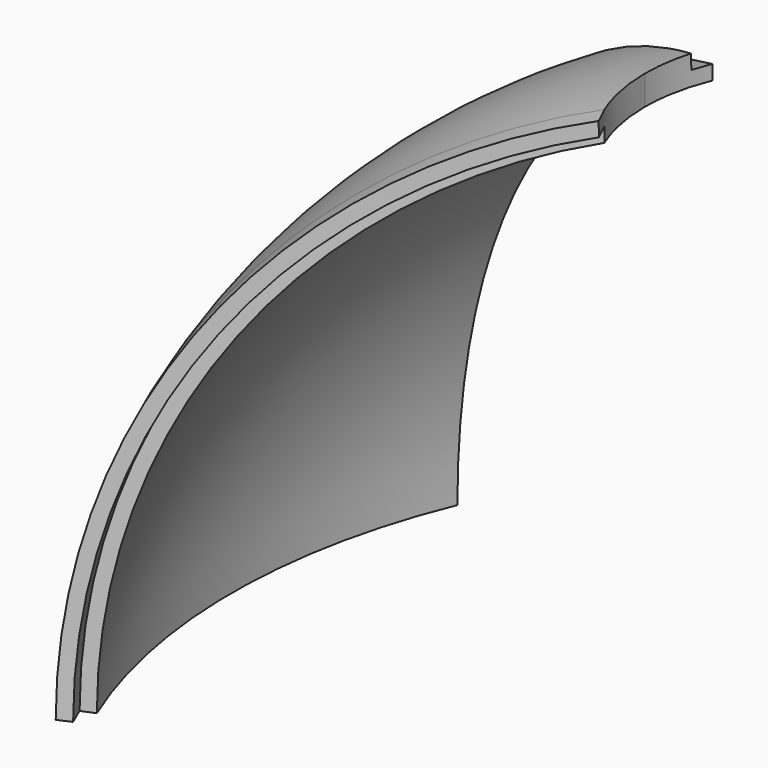
from build123d import *
from build123d import SkipClean  # not in build123d's __all__

# Parameters (mm, degrees)
F3_ANGLE_BACK = 22.5
F3_ANGLE      = 45
F8_W          = 1100
F8_H          = 4000


with BuildPart() as f3:
    # F2 (on Front) → F3 (revolve)
    with BuildSketch(Plane.XZ, mode=Mode.PRIVATE) as f3_sk:
        with BuildLine():
            Line((-1000, 3536.3293115885), (-1000, 3717.8622890043))
            ThreePointArc((-1000, 3717.8622890043), (-3055.5277776515, 2342.2745355743), (-3850, 0))
            Line((-3850, 0), (-3675, 0))
            ThreePointArc((-3675, 0), (-2930.9234892777, 2217.050405381), (-1000, 3536.3293115885))
        make_face()
    revolve(f3_sk.sketch.rotate(Axis((0, 0, 3762.5), (0, 0, 1)), -F3_ANGLE_BACK), axis=Axis((0, 0, 3762.5), (0, 0, 1)), revolution_arc=F3_ANGLE)

    # F5: sweep along a path in F5_path
    with BuildLine(Plane(origin=(-3556.9362001685, 1473.3312146056, 0), x_dir=(-0.9238795325, 0.3826834324, 0), z_dir=(-0.3826834324, -0.9238795325, 0))) as f5_path:
        ThreePointArc((0, 0), (-794.4722223485, -2342.2745355743), (-2850, -3717.8622890043))
    # F4 (on face) → F5 (sweep, cut)
    with BuildSketch(Plane(origin=(0, 0, 0), x_dir=(1, 0, 0), z_dir=(0, 0, -1))):
        with BuildLine():
            ThreePointArc((-3476.0967410737, -1439.8464142737), (-3498.6157300331, -1384.230552894), (-3520.2449580431, -1328.2626567709))
            Line((-3520.2449580431, -1328.2626567709), (-3602.111119858, -1359.1524859982))
            ThreePointArc((-3602.111119858, -1359.1524859982), (-3579.9788865455, -1416.4219611008), (-3556.9362001685, -1473.3312146056))
            Line((-3556.9362001685, -1473.3312146056), (-3476.0967410737, -1439.8464142737))
        make_face()
    sweep(path=f5_path.line, mode=Mode.SUBTRACT)

    # F7: sweep along a path in F7_path
    with BuildLine(Plane(origin=(-3556.9362001685, -1473.3312146056, 0), x_dir=(-0.9238795325, -0.3826834324, 0), z_dir=(0.3826834324, -0.9238795325, 0))) as f7_path:
        ThreePointArc((0, 0), (-794.4722223485, -2342.2745355743), (-2850, -3717.8622890043))
    # F6 (on face) → F7 (sweep)
    with BuildSketch(Plane(origin=(0, 0, 0), x_dir=(1, 0, 0), z_dir=(0, 0, -1))):
        with BuildLine():
            Line((-3428.4126130696, 1549.9655494704), (-3508.143138955, 1586.0112599232))
            ThreePointArc((-3508.143138955, 1586.0112599232), (-3532.9889208969, 1529.865773465), (-3556.9362001685, 1473.3312146056))
            Line((-3556.9362001685, 1473.3312146056), (-3476.0967410737, 1439.8464142737))
            ThreePointArc((-3476.0967410737, 1439.8464142736), (-3452.6937181493, 1495.0960967954), (-3428.4126130696, 1549.9655494704))
        make_face()
    with SkipClean():  # cleaning this boolean's faces spoils the solid; the shape is the same uncleaned
        sweep(path=f7_path.line)

    # F8 (on Front) → F9 (revolve, cut)
    with BuildSketch(Plane.XZ):
        with Locations((-550, 2000)):
            Rectangle(F8_W, F8_H)
    with SkipClean():  # cleaning this boolean's faces spoils the solid; the shape is the same uncleaned
        revolve(axis=Axis((0, 0, 2000), (0, 0, 1)), mode=Mode.SUBTRACT)


solid = f3.part
